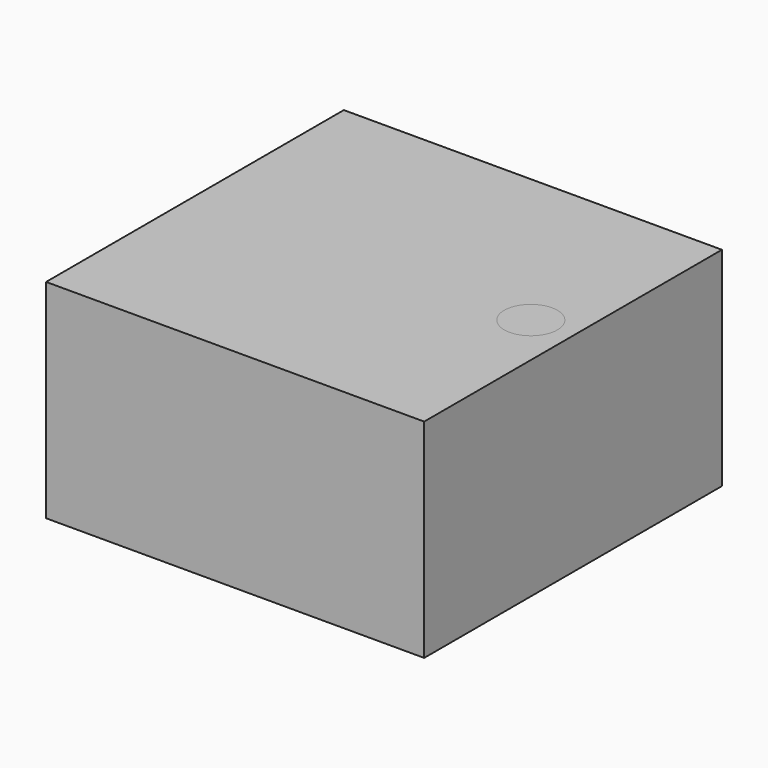
from build123d import *

# Parameters (mm, degrees)
F0_W     = 69.8630958796
F0_H     = 137.5265717506
F2_DEPTH = 76.8858
F1_R     = 9.8246353949


# Not quite as in the source:
# - the program builds the solid bodies; features that only make, move or delete a surface that nothing else refers to are left out


with BuildPart() as f2:
    # F0 (on Top) → F2 (new body)
    with BuildSketch(Plane.XY):
        with Locations((34.9315479398, 0)):
            Rectangle(F0_W, F0_H)
        with Locations((-34.9315479398, 0)):
            Rectangle(F0_W, F0_H)
    extrude(amount=F2_DEPTH)


with BuildPart() as f2b:
    # F1 (on Top) → F2, piece 2 (new body)
    with BuildSketch(Plane.XY):
        with Locations((54.2640089989, 0)):
            Circle(F1_R)
    extrude(amount=F2_DEPTH)


solid = Compound([f2.part, f2b.part])
